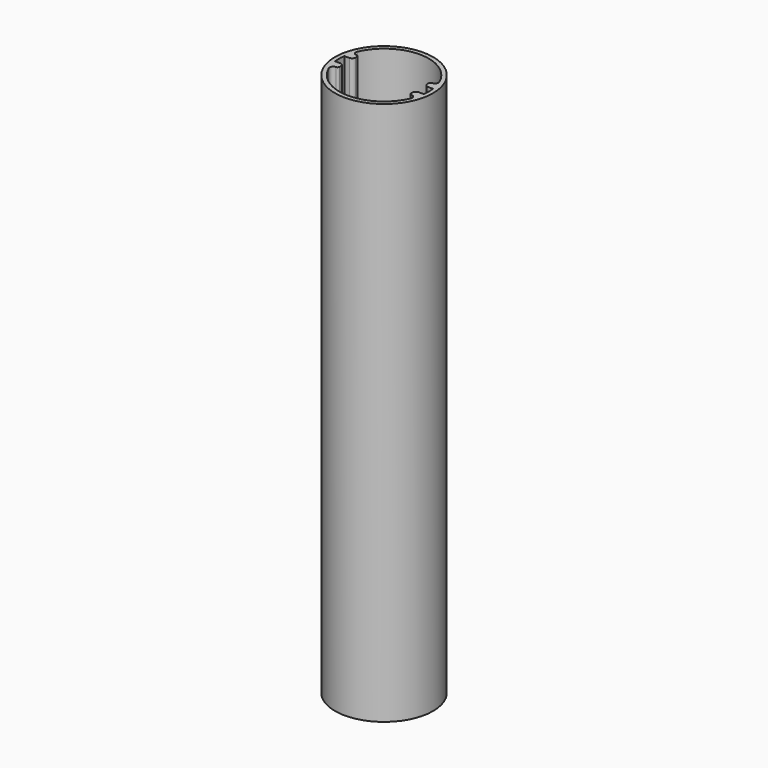
from build123d import *

# Parameters (mm, degrees)
F0_R           = 17.399
F0_R_2         = 3.175
F1_DEPTH       = 2.54
F2_R           = 5.461
F2_R_2         = 3.175
F3_DEPTH       = 3.81
F4_R           = 5.461
F4_R_2         = 3.937
F5_DEPTH       = 19.05
F6_R           = 17.399
F7_DEPTH       = 101.6
F9_DEPTH       = 30.48
F10_R          = 17.399
F11_DEPTH      = 88.9
F12_T1_DEPTH   = 25.1652142855
F12_T6_DEPTH   = 105.0543596926
F12_T11_DEPTH  = 104.2313774879
F12_T16_DEPTH  = 104.2313774879
F12_T21_DEPTH  = 105.4216753256
F12_T26_DEPTH  = 105.4216753256
F12_T31_DEPTH  = 105.4216753256
F12_T36_DEPTH  = 105.4216753256
F12_T41_DEPTH  = 104.2313774879
F12_T46_DEPTH  = 105.0543596926
F12_T51_DEPTH  = 104.2313774879
F12_T56_DEPTH  = 34.7565983231
F12_T61_DEPTH  = 34.7565983231
F12_T66_DEPTH  = 34.7565983231
F12_T71_DEPTH  = 34.7565983231
F12_T76_ANGLE  = 54.2466959693
F12_T82_ANGLE  = 54.2466959693
F12_T88_DEPTH  = 195.2350473194
F12_T93_DEPTH  = 195.2350473194
F12_T98_DEPTH  = 195.2350473194
F12_T103_DEPTH = 105.0543596926
F12_T108_DEPTH = 105.0543596926
F12_T113_DEPTH = 195.2350473194
F12_T119_DEPTH = 34.7565983231
F12_T123_ANGLE = 54.2466959693
F12_T130_ANGLE = 54.2466959693
F12_T134_DEPTH = 34.7565983231
F12_T141_DEPTH = 34.7565983231
F12_T145_ANGLE = 54.2466959693
F12_T152_ANGLE = 54.2466959693
F12_T156_DEPTH = 34.7565983231
F12_T159_DEPTH = 104.5853375167
F12_T161_DEPTH = 193.675
F13_R          = 0.762


# Not quite as in the source:
# - a fillet or chamfer that OpenCascade refuses, or shapes differently, is made with other operations: its cross-section is extruded or revolved along the edge and cut away or added


with BuildPart() as f1:
    # F0 (on Top) → F1 (new body)
    with BuildSketch(Plane.XY):
        Circle(F0_R)
        Circle(F0_R_2, mode=Mode.SUBTRACT)
    extrude(amount=F1_DEPTH)

    # F2 (on face) → F3 (join)
    with BuildSketch(Plane.XY.offset(2.54)):
        Circle(F2_R)
        Circle(F2_R_2, mode=Mode.SUBTRACT)
    extrude(amount=F3_DEPTH)

    # F4 (on face) → F5 (join)
    with BuildSketch(Plane.XY.offset(6.35)):
        Circle(F4_R)
        Circle(F4_R_2, mode=Mode.SUBTRACT)
    extrude(amount=F5_DEPTH)

    # F6 (on face) → F7 (join)
    with BuildSketch(Plane.XY.offset(2.54)):
        Circle(F6_R)
        with BuildLine():
            ThreePointArc((10.097205288, -12.2499824641), (0, -15.875), (-10.097205288, -12.2499824641))
            Line((-10.097205288, -12.2499824641), (-6.5712535066, -8.7240306827))
            ThreePointArc((-6.5712535066, -8.7240306827), (0, -10.922), (6.5712535066, -8.7240306827))
            Line((6.5712535066, -8.7240306827), (10.097205288, -12.2499824641))
        make_face(mode=Mode.SUBTRACT)
        with BuildLine():
            ThreePointArc((-15.2023827409, 4.572), (-13.6261710432, 8.1451266228), (-11.2253201513, 11.2253201513))
            Line((-11.2253201513, 11.2253201513), (-6.6453895296, 6.6453895296))
            ThreePointArc((-6.6453895296, 6.6453895296), (0, 9.398), (6.6453895296, 6.6453895296))
            Line((6.6453895296, 6.6453895296), (11.2253201513, 11.2253201513))
            ThreePointArc((11.2253201513, 11.2253201513), (13.6261710432, 8.1451266228), (15.2023827409, 4.572))
            Line((15.2023827409, 4.572), (12.7, 4.572))
            Line((12.7, 4.572), (12.7, 2.032))
            Line((12.7, 2.032), (15.7444149145, 2.032))
            ThreePointArc((15.7444149145, 2.032), (15.875, 0), (15.7444149145, -2.032))
            Line((15.7444149145, -2.032), (12.7, -2.032))
            Line((12.7, -2.032), (12.7, -4.572))
            Line((12.7, -4.572), (15.2023827409, -4.572))
            ThreePointArc((15.2023827409, -4.572), (13.6261710432, -8.1451266228), (11.2253201513, -11.2253201513))
            Line((11.2253201513, -11.2253201513), (6.6453895296, -6.6453895296))
            ThreePointArc((6.6453895296, -6.6453895296), (0, -9.398), (-6.6453895296, -6.6453895296))
            Line((-6.6453895296, -6.6453895296), (-11.2253201513, -11.2253201513))
            ThreePointArc((-11.2253201513, -11.2253201513), (-13.6261710432, -8.1451266228), (-15.2023827409, -4.572))
            Line((-15.2023827409, -4.572), (-12.7, -4.572))
            Line((-12.7, -4.572), (-12.7, -2.032))
            Line((-12.7, -2.032), (-15.7444149145, -2.032))
            ThreePointArc((-15.7444149145, -2.032), (-15.875, 0), (-15.7444149145, 2.032))
            Line((-15.7444149145, 2.032), (-12.7, 2.032))
            Line((-12.7, 2.032), (-12.7, 4.572))
            Line((-12.7, 4.572), (-15.2023827409, 4.572))
        make_face(mode=Mode.SUBTRACT)
        with BuildLine():
            Line((-6.5712535066, 8.7240306827), (-10.097205288, 12.2499824641))
            ThreePointArc((-10.097205288, 12.2499824641), (0, 15.875), (10.097205288, 12.2499824641))
            Line((10.097205288, 12.2499824641), (6.5712535066, 8.7240306827))
            ThreePointArc((6.5712535066, 8.7240306827), (0, 10.922), (-6.5712535066, 8.7240306827))
        make_face(mode=Mode.SUBTRACT)
    extrude(amount=F7_DEPTH)

    # F8 (on face) → F9 (join)
    with BuildSketch(Plane.XY.offset(2.54)):
        with BuildLine():
            ThreePointArc((1.27, 9.3117938122), (0, 9.398), (-1.27, 9.3117938122))
            Line((-1.27, 9.3117938122), (-1.27, 5.3112730112))
            ThreePointArc((-1.27, 5.3112730112), (0, 5.461), (1.27, 5.3112730112))
            Line((1.27, 5.3112730112), (1.27, 9.3117938122))
        make_face()
        with BuildLine():
            ThreePointArc((1.27, -5.3112730112), (0, -5.461), (-1.27, -5.3112730112))
            Line((-1.27, -5.3112730112), (-1.27, -9.3117938122))
            ThreePointArc((-1.27, -9.3117938122), (0, -9.398), (1.27, -9.3117938122))
            Line((1.27, -9.3117938122), (1.27, -5.3112730112))
        make_face()
    extrude(amount=F9_DEPTH)

    # F10 (on face) → F11 (join)
    with BuildSketch(Plane.XY.offset(104.14)):
        Circle(F10_R)
        with BuildLine():
            ThreePointArc((-15.2023827409, 4.572), (0, 15.875), (15.2023827409, 4.572))
            Line((15.2023827409, 4.572), (12.7, 4.572))
            Line((12.7, 4.572), (12.7, 2.032))
            Line((12.7, 2.032), (15.7444149145, 2.032))
            ThreePointArc((15.7444149145, 2.032), (15.875, 0), (15.7444149145, -2.032))
            Line((15.7444149145, -2.032), (12.7, -2.032))
            Line((12.7, -2.032), (12.7, -4.572))
            Line((12.7, -4.572), (15.2023827409, -4.572))
            ThreePointArc((15.2023827409, -4.572), (0, -15.875), (-15.2023827409, -4.572))
            Line((-15.2023827409, -4.572), (-12.7, -4.572))
            Line((-12.7, -4.572), (-12.7, -2.032))
            Line((-12.7, -2.032), (-15.7444149145, -2.032))
            ThreePointArc((-15.7444149145, -2.032), (-15.875, 0), (-15.7444149145, 2.032))
            Line((-15.7444149145, 2.032), (-12.7, 2.032))
            Line((-12.7, 2.032), (-12.7, 4.572))
            Line((-12.7, 4.572), (-15.2023827409, 4.572))
        make_face(mode=Mode.SUBTRACT)
    extrude(amount=F11_DEPTH)

    # F12: fillet of radius 1.27 on 34 edges, made by hand

    # F12_s2 → F12_t1 (join)
    with BuildSketch(Plane.XY.offset(0.2347857145)):
        with BuildLine():
            ThreePointArc((1.27, 6.2333587254), (1.4860689042, 5.52474794), (2.060754717, 5.0572533055))
            ThreePointArc((2.060754717, 5.0572533055), (1.6702135339, 5.1993180083), (1.27, 5.3112730112))
            Line((1.27, 5.3112730112), (1.27, 6.2333587254))
        make_face()
        with BuildLine():
            ThreePointArc((1.27, -6.2333587254), (1.4860689042, -5.52474794), (2.060754717, -5.0572533055))
            ThreePointArc((2.060754717, -5.0572533055), (1.6702135339, -5.1993180083), (1.27, -5.3112730112))
            Line((1.27, -5.3112730112), (1.27, -6.2333587254))
        make_face()
        with BuildLine():
            ThreePointArc((-2.060754717, 5.0572533055), (-1.4860689042, 5.52474794), (-1.27, 6.2333587254))
            Line((-1.27, 6.2333587254), (-1.27, 5.3112730112))
            ThreePointArc((-1.27, 5.3112730112), (-1.6702135339, 5.1993180083), (-2.060754717, 5.0572533055))
        make_face()
        with BuildLine():
            ThreePointArc((-1.27, -6.2333587254), (-1.4860689042, -5.52474794), (-2.060754717, -5.0572533055))
            ThreePointArc((-2.060754717, -5.0572533055), (-1.6702135339, -5.1993180083), (-1.27, -5.3112730112))
            Line((-1.27, -5.3112730112), (-1.27, -6.2333587254))
        make_face()
    extrude(amount=F12_T1_DEPTH)


with BuildPart() as f12_tool4:
    # F12_s5 → F12_t6 (new body)
    with BuildSketch(Plane.XY.offset(-0.9143596926)):
        with BuildLine():
            ThreePointArc((10.2881758587, -10.2881758587), (11.2414712259, -10.6589470208), (12.1589146422, -10.2066850507))
            ThreePointArc((12.1589146422, -10.2066850507), (11.7032052698, -10.7261648045), (11.2253201513, -11.2253201513))
            Line((11.2253201513, -11.2253201513), (10.2881758587, -10.2881758587))
        make_face()
    extrude(amount=F12_T6_DEPTH)

    split(bisect_by=Plane.XY, keep=Keep.TOP)


with BuildPart() as f1_1:
    add(f1.part)

    # F12_t3: union F12_tool4
    add(f12_tool4.part)


with BuildPart() as f12_tool9:
    # F12_s10 → F12_t11 (new body)
    with BuildSketch(Plane.XY.offset(-0.0913774879)):
        with BuildLine():
            ThreePointArc((-7.3155194528, -9.4682966289), (-6.5638992584, -9.1047892634), (-5.749004899, -9.2864970076))
            ThreePointArc((-5.749004899, -9.2864970076), (-6.1665455392, -9.0146436487), (-6.5712535066, -8.7240306827))
            Line((-6.5712535066, -8.7240306827), (-7.3155194528, -9.4682966289))
        make_face()
    extrude(amount=F12_T11_DEPTH)

    split(bisect_by=Plane.XY, keep=Keep.TOP)


with BuildPart() as f1_2:
    add(f1_1.part)

    # F12_t8: union F12_tool9
    add(f12_tool9.part)


with BuildPart() as f12_tool14:
    # F12_s15 → F12_t16 (new body)
    with BuildSketch(Plane.XY.offset(-0.0913774879)):
        with BuildLine():
            ThreePointArc((5.749004899, -9.2864970076), (6.5638992584, -9.1047892634), (7.3155194528, -9.4682966289))
            Line((7.3155194528, -9.4682966289), (6.5712535066, -8.7240306827))
            ThreePointArc((6.5712535066, -8.7240306827), (6.1665455392, -9.0146436487), (5.749004899, -9.2864970076))
        make_face()
    extrude(amount=F12_T16_DEPTH)

    split(bisect_by=Plane.XY, keep=Keep.TOP)


with BuildPart() as f1_3:
    add(f1_2.part)

    # F12_t13: union F12_tool14
    add(f12_tool14.part)


with BuildPart() as f12_tool19:
    # F12_s20 → F12_t21 (new body)
    with BuildSketch(Plane.XY.offset(-1.2816753256)):
        with BuildLine():
            ThreePointArc((9.0604107622, -11.2131879382), (9.426515043, -12.2331791758), (8.8721577718, -13.1643625547))
            ThreePointArc((8.8721577718, -13.1643625547), (9.4956941011, -12.7219266834), (10.097205288, -12.2499824641))
            Line((10.097205288, -12.2499824641), (9.0604107622, -11.2131879382))
        make_face()
    extrude(amount=F12_T21_DEPTH)

    split(bisect_by=Plane.XY, keep=Keep.TOP)


with BuildPart() as f1_4:
    add(f1_3.part)

    # F12_t18: union F12_tool19
    add(f12_tool19.part)


with BuildPart() as f12_tool24:
    # F12_s25 → F12_t26 (new body)
    with BuildSketch(Plane.XY.offset(-1.2816753256)):
        with BuildLine():
            ThreePointArc((-9.0604107622, -11.2131879382), (-9.426515043, -12.2331791758), (-8.8721577718, -13.1643625547))
            ThreePointArc((-8.8721577718, -13.1643625547), (-9.4956941011, -12.7219266834), (-10.097205288, -12.2499824641))
            Line((-10.097205288, -12.2499824641), (-9.0604107622, -11.2131879382))
        make_face()
    extrude(amount=F12_T26_DEPTH)

    split(bisect_by=Plane.XY, keep=Keep.TOP)


with BuildPart() as f1_5:
    add(f1_4.part)

    # F12_t23: union F12_tool24
    add(f12_tool24.part)


with BuildPart() as f12_tool29:
    # F12_s30 → F12_t31 (new body)
    with BuildSketch(Plane.XY.offset(-1.2816753256)):
        with BuildLine():
            ThreePointArc((-9.0604107622, 11.2131879382), (-9.426515043, 12.2331791758), (-8.8721577718, 13.1643625547))
            ThreePointArc((-8.8721577718, 13.1643625547), (-9.4956941011, 12.7219266834), (-10.097205288, 12.2499824641))
            Line((-10.097205288, 12.2499824641), (-9.0604107622, 11.2131879382))
        make_face()
    extrude(amount=F12_T31_DEPTH)

    split(bisect_by=Plane.XY, keep=Keep.TOP)


with BuildPart() as f1_6:
    add(f1_5.part)

    # F12_t28: union F12_tool29
    add(f12_tool29.part)


with BuildPart() as f12_tool34:
    # F12_s35 → F12_t36 (new body)
    with BuildSketch(Plane.XY.offset(-1.2816753256)):
        with BuildLine():
            ThreePointArc((9.0604107622, 11.2131879382), (9.426515043, 12.2331791758), (8.8721577718, 13.1643625547))
            ThreePointArc((8.8721577718, 13.1643625547), (9.4956941011, 12.7219266834), (10.097205288, 12.2499824641))
            Line((10.097205288, 12.2499824641), (9.0604107622, 11.2131879382))
        make_face()
    extrude(amount=F12_T36_DEPTH)

    split(bisect_by=Plane.XY, keep=Keep.TOP)


with BuildPart() as f1_7:
    add(f1_6.part)

    # F12_t33: union F12_tool34
    add(f12_tool34.part)


with BuildPart() as f12_tool39:
    # F12_s40 → F12_t41 (new body)
    with BuildSketch(Plane.XY.offset(-0.0913774879)):
        with BuildLine():
            ThreePointArc((7.3155194528, 9.4682966289), (6.5638992584, 9.1047892634), (5.749004899, 9.2864970076))
            ThreePointArc((5.749004899, 9.2864970076), (6.1665455392, 9.0146436487), (6.5712535066, 8.7240306827))
            Line((6.5712535066, 8.7240306827), (7.3155194528, 9.4682966289))
        make_face()
    extrude(amount=F12_T41_DEPTH)

    split(bisect_by=Plane.XY, keep=Keep.TOP)


with BuildPart() as f1_8:
    add(f1_7.part)

    # F12_t38: union F12_tool39
    add(f12_tool39.part)


with BuildPart() as f12_tool44:
    # F12_s45 → F12_t46 (new body)
    with BuildSketch(Plane.XY.offset(-0.9143596926)):
        with BuildLine():
            ThreePointArc((-10.2881758587, 10.2881758587), (-11.2414712259, 10.6589470208), (-12.1589146422, 10.2066850507))
            ThreePointArc((-12.1589146422, 10.2066850507), (-11.7032052698, 10.7261648045), (-11.2253201513, 11.2253201513))
            Line((-11.2253201513, 11.2253201513), (-10.2881758587, 10.2881758587))
        make_face()
    extrude(amount=F12_T46_DEPTH)

    split(bisect_by=Plane.XY, keep=Keep.TOP)


with BuildPart() as f1_9:
    add(f1_8.part)

    # F12_t43: union F12_tool44
    add(f12_tool44.part)


with BuildPart() as f12_tool49:
    # F12_s50 → F12_t51 (new body)
    with BuildSketch(Plane.XY.offset(-0.0913774879)):
        with BuildLine():
            ThreePointArc((-5.749004899, 9.2864970076), (-6.5638992584, 9.1047892634), (-7.3155194528, 9.4682966289))
            Line((-7.3155194528, 9.4682966289), (-6.5712535066, 8.7240306827))
            ThreePointArc((-6.5712535066, 8.7240306827), (-6.1665455392, 9.0146436487), (-5.749004899, 9.2864970076))
        make_face()
    extrude(amount=F12_T51_DEPTH)

    split(bisect_by=Plane.XY, keep=Keep.TOP)


with BuildPart() as f1_10:
    add(f1_9.part)

    # F12_t48: union F12_tool49
    add(f12_tool49.part)


with BuildPart() as f12_tool54:
    # F12_s55 → F12_t56 (new body)
    with BuildSketch(Plane.XY.offset(-1.7365983231)):
        with BuildLine():
            ThreePointArc((1.27, 7.72093155), (1.7953964981, 8.7497491359), (2.936875, 8.9273271047))
            ThreePointArc((2.936875, 8.9273271047), (2.1122033469, 9.1575652343), (1.27, 9.3117938122))
            Line((1.27, 9.3117938122), (1.27, 7.72093155))
        make_face()
    extrude(amount=F12_T56_DEPTH)

    split(bisect_by=Plane.XY, keep=Keep.TOP)


with BuildPart() as f1_11:
    add(f1_10.part)

    # F12_t53: union F12_tool54
    add(f12_tool54.part)


with BuildPart() as f12_tool59:
    # F12_s60 → F12_t61 (new body)
    with BuildSketch(Plane.XY.offset(-1.7365983231)):
        with BuildLine():
            ThreePointArc((1.27, -7.72093155), (1.7953964981, -8.7497491359), (2.936875, -8.9273271047))
            ThreePointArc((2.936875, -8.9273271047), (2.1122033469, -9.1575652343), (1.27, -9.3117938122))
            Line((1.27, -9.3117938122), (1.27, -7.72093155))
        make_face()
    extrude(amount=F12_T61_DEPTH)

    split(bisect_by=Plane.XY, keep=Keep.TOP)


with BuildPart() as f1_12:
    add(f1_11.part)

    # F12_t58: union F12_tool59
    add(f12_tool59.part)


with BuildPart() as f12_tool64:
    # F12_s65 → F12_t66 (new body)
    with BuildSketch(Plane.XY.offset(-1.7365983231)):
        with BuildLine():
            ThreePointArc((-1.27, -7.72093155), (-1.7953964981, -8.7497491359), (-2.936875, -8.9273271047))
            ThreePointArc((-2.936875, -8.9273271047), (-2.1122033469, -9.1575652343), (-1.27, -9.3117938122))
            Line((-1.27, -9.3117938122), (-1.27, -7.72093155))
        make_face()
    extrude(amount=F12_T66_DEPTH)

    split(bisect_by=Plane.XY, keep=Keep.TOP)


with BuildPart() as f1_13:
    add(f1_12.part)

    # F12_t63: union F12_tool64
    add(f12_tool64.part)


with BuildPart() as f12_tool69:
    # F12_s70 → F12_t71 (new body)
    with BuildSketch(Plane.XY.offset(-1.7365983231)):
        with BuildLine():
            ThreePointArc((-1.27, 7.72093155), (-1.7953964981, 8.7497491359), (-2.936875, 8.9273271047))
            ThreePointArc((-2.936875, 8.9273271047), (-2.1122033469, 9.1575652343), (-1.27, 9.3117938122))
            Line((-1.27, 9.3117938122), (-1.27, 7.72093155))
        make_face()
    extrude(amount=F12_T71_DEPTH)

    split(bisect_by=Plane.XY, keep=Keep.TOP)


with BuildPart() as f1_14:
    add(f1_13.part)

    # F12_t68: union F12_tool69
    add(f12_tool69.part)


with BuildPart() as f12_tool74:
    # F12_s75 → F12_t76 (revolve)
    with BuildSketch(Plane(origin=(0, 0, 0), x_dir=(0, 0, 1), z_dir=(0.8900270965, -0.4559076304, 0))):
        with BuildLine():
            ThreePointArc((33.02, -8.128), (33.3919743879, -9.0260256121), (34.29, -9.398))
            Line((34.29, -9.398), (33.02, -9.398))
            Line((33.02, -9.398), (33.02, -8.128))
        make_face()
    revolve(axis=Axis((0, 0, 33.02), (0, 0, 1)), revolution_arc=F12_T76_ANGLE)

    split(bisect_by=Plane.YZ.offset(1.27), keep=Keep.BOTTOM)

    split(bisect_by=Plane.YZ.offset(-1.27), keep=Keep.TOP)


with BuildPart() as f1_15:
    add(f1_14.part)

    # F12_t73: union F12_tool74
    add(f12_tool74.part)


with BuildPart() as f12_tool80:
    # F12_s81 → F12_t82 (revolve)
    with BuildSketch(Plane(origin=(0, 0, 0), x_dir=(0, 0, 1), z_dir=(-0.8900270965, 0.4559076304, 0))):
        with BuildLine():
            ThreePointArc((33.02, -8.128), (33.3919743879, -9.0260256121), (34.29, -9.398))
            Line((34.29, -9.398), (33.02, -9.398))
            Line((33.02, -9.398), (33.02, -8.128))
        make_face()
    revolve(axis=Axis((0, 0, 33.02), (0, 0, 1)), revolution_arc=F12_T82_ANGLE)

    split(bisect_by=Plane.YZ.offset(-1.27), keep=Keep.TOP)

    split(bisect_by=Plane.YZ.offset(1.27), keep=Keep.BOTTOM)


with BuildPart() as f1_16:
    add(f1_15.part)

    # F12_t79: union F12_tool80
    add(f12_tool80.part)


with BuildPart() as f12_tool86:
    # F12_s87 → F12_t88 (new body)
    with BuildSketch(Plane.XY.offset(-2.1950473194)):
        with BuildLine():
            ThreePointArc((-13.385703605, -4.572), (-14.4482618387, -5.146392352), (-14.5496778315, -6.35))
            ThreePointArc((-14.5496778315, -6.35), (-14.9025701835, -5.4707428129), (-15.2023827409, -4.572))
            Line((-15.2023827409, -4.572), (-13.385703605, -4.572))
        make_face()
    extrude(amount=F12_T88_DEPTH)

    split(bisect_by=Plane.XY, keep=Keep.TOP)


with BuildPart() as f1_17:
    add(f1_16.part)

    # F12_t85: union F12_tool86
    add(f12_tool86.part)


with BuildPart() as f12_tool91:
    # F12_s92 → F12_t93 (new body)
    with BuildSketch(Plane.XY.offset(-2.1950473194)):
        with BuildLine():
            ThreePointArc((13.385703605, 4.572), (14.4482618387, 5.146392352), (14.5496778315, 6.35))
            ThreePointArc((14.5496778315, 6.35), (14.9025701835, 5.4707428129), (15.2023827409, 4.572))
            Line((15.2023827409, 4.572), (13.385703605, 4.572))
        make_face()
    extrude(amount=F12_T93_DEPTH)

    split(bisect_by=Plane.XY, keep=Keep.TOP)


with BuildPart() as f1_18:
    add(f1_17.part)

    # F12_t90: union F12_tool91
    add(f12_tool91.part)


with BuildPart() as f12_tool96:
    # F12_s97 → F12_t98 (new body)
    with BuildSketch(Plane.XY.offset(193.04)):
        with BuildLine():
            ThreePointArc((-13.385703605, 4.572), (-14.4482618387, 5.146392352), (-14.5496778315, 6.35))
            ThreePointArc((-14.5496778315, 6.35), (-14.9025701835, 5.4707428129), (-15.2023827409, 4.572))
            Line((-15.2023827409, 4.572), (-13.385703605, 4.572))
        make_face()
    extrude(amount=-F12_T98_DEPTH)

    split(bisect_by=Plane.XY, keep=Keep.TOP)


with BuildPart() as f1_19:
    add(f1_18.part)

    # F12_t95: union F12_tool96
    add(f12_tool96.part)


with BuildPart() as f12_tool101:
    # F12_s102 → F12_t103 (new body)
    with BuildSketch(Plane.XY.offset(-0.9143596926)):
        with BuildLine():
            ThreePointArc((10.2881758587, 10.2881758587), (11.2414712259, 10.6589470208), (12.1589146422, 10.2066850507))
            ThreePointArc((12.1589146422, 10.2066850507), (11.7032052698, 10.7261648045), (11.2253201513, 11.2253201513))
            Line((11.2253201513, 11.2253201513), (10.2881758587, 10.2881758587))
        make_face()
    extrude(amount=F12_T103_DEPTH)

    split(bisect_by=Plane.XY, keep=Keep.TOP)


with BuildPart() as f1_20:
    add(f1_19.part)

    # F12_t100: union F12_tool101
    add(f12_tool101.part)


with BuildPart() as f12_tool106:
    # F12_s107 → F12_t108 (new body)
    with BuildSketch(Plane.XY.offset(-0.9143596926)):
        with BuildLine():
            ThreePointArc((-10.2881758587, -10.2881758587), (-11.2414712259, -10.6589470208), (-12.1589146422, -10.2066850507))
            ThreePointArc((-12.1589146422, -10.2066850507), (-11.7032052698, -10.7261648045), (-11.2253201513, -11.2253201513))
            Line((-11.2253201513, -11.2253201513), (-10.2881758587, -10.2881758587))
        make_face()
    extrude(amount=F12_T108_DEPTH)

    split(bisect_by=Plane.XY, keep=Keep.TOP)


with BuildPart() as f1_21:
    add(f1_20.part)

    # F12_t105: union F12_tool106
    add(f12_tool106.part)


with BuildPart() as f12_tool111:
    # F12_s112 → F12_t113 (new body)
    with BuildSketch(Plane.XY.offset(-2.1950473194)):
        with BuildLine():
            ThreePointArc((14.5496778315, -6.35), (14.4482618387, -5.146392352), (13.385703605, -4.572))
            Line((13.385703605, -4.572), (15.2023827409, -4.572))
            ThreePointArc((15.2023827409, -4.572), (14.9025701835, -5.4707428129), (14.5496778315, -6.35))
        make_face()
    extrude(amount=F12_T113_DEPTH)

    split(bisect_by=Plane.XY, keep=Keep.TOP)


with BuildPart() as f1_22:
    add(f1_21.part)

    # F12_t110: union F12_tool111
    add(f12_tool111.part)


with BuildPart() as f12_tool117:
    # F12_s118 → F12_t119 (new body)
    with BuildSketch(Plane.XY.offset(2.54)):
        with BuildLine():
            ThreePointArc((1.27, 7.72093155), (1.7953964981, 8.7497491359), (2.936875, 8.9273271047))
            ThreePointArc((2.936875, 8.9273271047), (2.1122033469, 9.1575652343), (1.27, 9.3117938122))
            Line((1.27, 9.3117938122), (1.27, 7.72093155))
        make_face()
    extrude(amount=F12_T119_DEPTH)

    split(bisect_by=Plane.XY.offset(33.02), keep=Keep.TOP)


with BuildPart() as f12_tool121:
    # F12_s122 → F12_t123 (revolve)
    with BuildSketch(Plane(origin=(0, 0, 0), x_dir=(0, 0, 1), z_dir=(0.8900270965, -0.4559076304, 0))):
        with BuildLine():
            ThreePointArc((33.02, -8.128), (33.3919743879, -9.0260256121), (34.29, -9.398))
            Line((34.29, -9.398), (33.02, -9.398))
            Line((33.02, -9.398), (33.02, -8.128))
        make_face()
    revolve(axis=Axis((0, 0, 33.02), (0, 0, 1)), revolution_arc=F12_T123_ANGLE)

    split(bisect_by=Plane.YZ.offset(1.27), keep=Keep.TOP)


with BuildPart() as f12_tool117_1:
    add(f12_tool117.part)

    # F12_t125: intersect F12_tool121
    add(f12_tool121.part, mode=Mode.INTERSECT)


with BuildPart() as f1_23:
    add(f1_22.part)

    # F12_t115: union F12_tool117
    add(f12_tool117_1.part)


with BuildPart() as f12_tool128:
    # F12_s129 → F12_t130 (revolve)
    with BuildSketch(Plane(origin=(0, 0, 0), x_dir=(0, 0, 1), z_dir=(-0.8900270965, 0.4559076304, 0))):
        with BuildLine():
            ThreePointArc((33.02, -8.128), (33.3919743879, -9.0260256121), (34.29, -9.398))
            Line((34.29, -9.398), (33.02, -9.398))
            Line((33.02, -9.398), (33.02, -8.128))
        make_face()
    revolve(axis=Axis((0, 0, 33.02), (0, 0, 1)), revolution_arc=F12_T130_ANGLE)

    split(bisect_by=Plane.YZ.offset(1.27), keep=Keep.TOP)


with BuildPart() as f12_tool132:
    # F12_s133 → F12_t134 (new body)
    with BuildSketch(Plane.XY.offset(2.54)):
        with BuildLine():
            ThreePointArc((1.27, -7.72093155), (1.7953964981, -8.7497491359), (2.936875, -8.9273271047))
            ThreePointArc((2.936875, -8.9273271047), (2.1122033469, -9.1575652343), (1.27, -9.3117938122))
            Line((1.27, -9.3117938122), (1.27, -7.72093155))
        make_face()
    extrude(amount=F12_T134_DEPTH)

    split(bisect_by=Plane.XY.offset(33.02), keep=Keep.TOP)


with BuildPart() as f12_tool128_1:
    add(f12_tool128.part)

    # F12_t136: intersect F12_tool132
    add(f12_tool132.part, mode=Mode.INTERSECT)


with BuildPart() as f1_24:
    add(f1_23.part)

    # F12_t126: union F12_tool128
    add(f12_tool128_1.part)


with BuildPart() as f12_tool139:
    # F12_s140 → F12_t141 (new body)
    with BuildSketch(Plane.XY.offset(2.54)):
        with BuildLine():
            ThreePointArc((-1.27, -7.72093155), (-1.7953964981, -8.7497491359), (-2.936875, -8.9273271047))
            ThreePointArc((-2.936875, -8.9273271047), (-2.1122033469, -9.1575652343), (-1.27, -9.3117938122))
            Line((-1.27, -9.3117938122), (-1.27, -7.72093155))
        make_face()
    extrude(amount=F12_T141_DEPTH)

    split(bisect_by=Plane.XY.offset(33.02), keep=Keep.TOP)


with BuildPart() as f12_tool143:
    # F12_s144 → F12_t145 (revolve)
    with BuildSketch(Plane(origin=(0, 0, 0), x_dir=(0, 0, 1), z_dir=(-0.8900270965, 0.4559076304, 0))):
        with BuildLine():
            ThreePointArc((33.02, -8.128), (33.3919743879, -9.0260256121), (34.29, -9.398))
            Line((34.29, -9.398), (33.02, -9.398))
            Line((33.02, -9.398), (33.02, -8.128))
        make_face()
    revolve(axis=Axis((0, 0, 33.02), (0, 0, 1)), revolution_arc=F12_T145_ANGLE)

    split(bisect_by=Plane.YZ.offset(-1.27), keep=Keep.BOTTOM)


with BuildPart() as f12_tool139_1:
    add(f12_tool139.part)

    # F12_t147: intersect F12_tool143
    add(f12_tool143.part, mode=Mode.INTERSECT)


with BuildPart() as f1_25:
    add(f1_24.part)

    # F12_t137: union F12_tool139
    add(f12_tool139_1.part)


with BuildPart() as f12_tool150:
    # F12_s151 → F12_t152 (revolve)
    with BuildSketch(Plane(origin=(0, 0, 0), x_dir=(0, 0, 1), z_dir=(0.8900270965, -0.4559076304, 0))):
        with BuildLine():
            ThreePointArc((33.02, -8.128), (33.3919743879, -9.0260256121), (34.29, -9.398))
            Line((34.29, -9.398), (33.02, -9.398))
            Line((33.02, -9.398), (33.02, -8.128))
        make_face()
    revolve(axis=Axis((0, 0, 33.02), (0, 0, 1)), revolution_arc=F12_T152_ANGLE)

    split(bisect_by=Plane.YZ.offset(-1.27), keep=Keep.BOTTOM)


with BuildPart() as f12_tool154:
    # F12_s155 → F12_t156 (new body)
    with BuildSketch(Plane.XY.offset(2.54)):
        with BuildLine():
            ThreePointArc((-1.27, 7.72093155), (-1.7953964981, 8.7497491359), (-2.936875, 8.9273271047))
            ThreePointArc((-2.936875, 8.9273271047), (-2.1122033469, 9.1575652343), (-1.27, 9.3117938122))
            Line((-1.27, 9.3117938122), (-1.27, 7.72093155))
        make_face()
    extrude(amount=F12_T156_DEPTH)

    split(bisect_by=Plane.XY.offset(33.02), keep=Keep.TOP)


with BuildPart() as f12_tool150_1:
    add(f12_tool150.part)

    # F12_t158: intersect F12_tool154
    add(f12_tool154.part, mode=Mode.INTERSECT)


with BuildPart() as f1_26:
    add(f1_25.part)

    # F12_t148: union F12_tool150
    add(f12_tool150_1.part)

    # F12_s160 → F12_t159 (cut)
    with BuildSketch(Plane.XY.offset(2.54)):
        with BuildLine():
            ThreePointArc((-7.4897704905, -7.4897704905), (-6.667474874, -7.120056), (-5.8070133452, -7.3892489475))
            ThreePointArc((-5.8070133452, -7.3892489475), (-6.2373003814, -7.029828444), (-6.6453895296, -6.6453895296))
            Line((-6.6453895296, -6.6453895296), (-7.4897704905, -7.4897704905))
        make_face()
        with BuildLine():
            ThreePointArc((7.4897704905, -7.4897704905), (6.667474874, -7.120056), (5.8070133452, -7.3892489475))
            ThreePointArc((5.8070133452, -7.3892489475), (6.2373003814, -7.029828444), (6.6453895296, -6.6453895296))
            Line((6.6453895296, -6.6453895296), (7.4897704905, -7.4897704905))
        make_face()
        with BuildLine():
            ThreePointArc((-5.8070133452, 7.3892489475), (-6.667474874, 7.120056), (-7.4897704905, 7.4897704905))
            Line((-7.4897704905, 7.4897704905), (-6.6453895296, 6.6453895296))
            ThreePointArc((-6.6453895296, 6.6453895296), (-6.2373003814, 7.029828444), (-5.8070133452, 7.3892489475))
        make_face()
        with BuildLine():
            ThreePointArc((7.4897704905, 7.4897704905), (6.667474874, 7.120056), (5.8070133452, 7.3892489475))
            ThreePointArc((5.8070133452, 7.3892489475), (6.2373003814, 7.029828444), (6.6453895296, 6.6453895296))
            Line((6.6453895296, 6.6453895296), (7.4897704905, 7.4897704905))
        make_face()
    extrude(amount=F12_T159_DEPTH, mode=Mode.SUBTRACT)

    # F12_s162 → F12_t161 (cut)
    with BuildSketch(Plane.XY.offset(2.54)):
        with BuildLine():
            ThreePointArc((-12.7, 3.302), (-13.0719743879, 2.4039743879), (-13.97, 2.032))
            Line((-13.97, 2.032), (-12.7, 2.032))
            Line((-12.7, 2.032), (-12.7, 3.302))
        make_face()
        with BuildLine():
            ThreePointArc((-13.97, -2.032), (-13.0719743879, -2.4039743879), (-12.7, -3.302))
            Line((-12.7, -3.302), (-12.7, -2.032))
            Line((-12.7, -2.032), (-13.97, -2.032))
        make_face()
        with BuildLine():
            ThreePointArc((13.97, 2.032), (13.0719743879, 2.4039743879), (12.7, 3.302))
            Line((12.7, 3.302), (12.7, 2.032))
            Line((12.7, 2.032), (13.97, 2.032))
        make_face()
        with BuildLine():
            ThreePointArc((12.7, -3.302), (13.0719743879, -2.4039743879), (13.97, -2.032))
            Line((13.97, -2.032), (12.7, -2.032))
            Line((12.7, -2.032), (12.7, -3.302))
        make_face()
    extrude(amount=F12_T161_DEPTH, mode=Mode.SUBTRACT)

    # F13
    f13_edges = [f1_26.edges().sort_by_distance(p)[0] for p in [
        (-12.7, -4.572, 97.79),
        (-12.7, 4.572, 97.79),
        (12.7, 4.572, 97.79),
        (12.7, -4.572, 97.79),
    ]]
    fillet(f13_edges, radius=F13_R)


solid = f1_26.part
